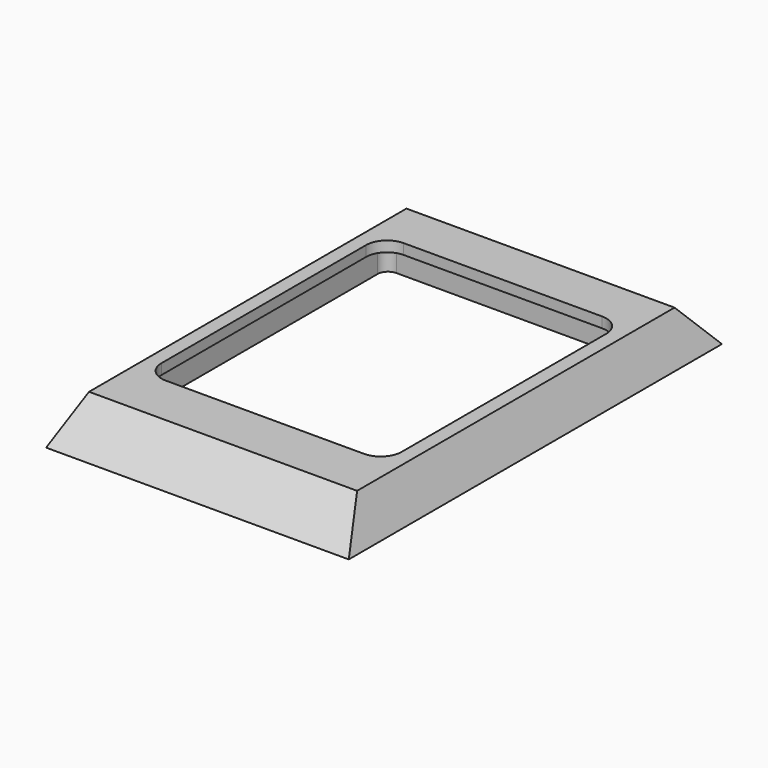
from build123d import *

# Parameters (mm, degrees)
F1_W        = 60
F1_H        = 93
F2_DEPTH    = 8
F3_T1_DEPTH = 147.142599219
F4_T1_DEPTH = 102.8305675527
F5_DEPTH    = 25
F6_DEPTH    = 6
F7_T1_DEPTH = 105.1482614058


# Not quite as in the source:
# - a fillet or chamfer that OpenCascade refuses, or shapes differently, is made with other operations: its cross-section is extruded or revolved along the edge and cut away or added


with BuildPart() as f2:
    # F1 (on Top) → F2 (new body)
    with BuildSketch(Plane.XY):
        Rectangle(F1_W, F1_H)
    extrude(amount=F2_DEPTH)

    # F3: chamfer of 4.325 x 10.4414736573 on 2 edges, made by hand

    # F3_s2 → F3_t1 (cut)
    with BuildSketch(Plane.XZ.offset(-73.5712996095)):
        Polygon((30, -2.4414736573), (25.675, 8), (30, 8), align=None)
        Polygon((-30, -2.4414736573), (-25.675, 8), (-30, 8), align=None)
    extrude(amount=F3_T1_DEPTH, mode=Mode.SUBTRACT)

    # F4: chamfer of 9 x 9.9955126335 on 1 edges, made by hand

    # F4_s2 → F4_t1 (cut)
    with BuildSketch(Plane.YZ.offset(-51.4152837764)):
        Polygon((37.5, 8), (46.5, -1.9955126335), (46.5, 8), align=None)
    extrude(amount=F4_T1_DEPTH, mode=Mode.SUBTRACT)

    # F0 (on Top) → F5 (cut)
    with BuildSketch(Plane.XY):
        with BuildLine():
            ThreePointArc((23, 24.5), (21.8284271247, 27.3284271247), (19, 28.5))
            Line((19, 28.5), (-19, 28.5))
            ThreePointArc((-19, 28.5), (-21.8284271247, 27.3284271247), (-23, 24.5))
            Line((-23, 24.5), (-23, -24.5))
            ThreePointArc((-23, -24.5), (-21.8284271247, -27.3284271247), (-19, -28.5))
            Line((-19, -28.5), (19, -28.5))
            ThreePointArc((19, -28.5), (21.8284271247, -27.3284271247), (23, -24.5))
            Line((23, -24.5), (23, 24.5))
        make_face()
    extrude(amount=F5_DEPTH, mode=Mode.SUBTRACT)

    # F0 (on Top) → F6 (cut)
    with BuildSketch(Plane.XY):
        with BuildLine():
            ThreePointArc((25.6034387499, 30.25), (25.0176523123, 31.6642135624), (23.6034387499, 32.25))
            Line((23.6034387499, 32.25), (-23.3965612501, 32.25))
            ThreePointArc((-23.3965612501, 32.25), (-24.8107748125, 31.6642135624), (-25.3965612501, 30.25))
            Line((-25.3965612501, 30.25), (-25.3965612501, -35.75))
            ThreePointArc((-25.3965612501, -35.75), (-24.8107748125, -37.1642135624), (-23.3965612501, -37.75))
            Line((-23.3965612501, -37.75), (23.6034387499, -37.75))
            ThreePointArc((23.6034387499, -37.75), (25.0176523123, -37.1642135624), (25.6034387499, -35.75))
            Line((25.6034387499, -35.75), (25.6034387499, 30.25))
        make_face()
        with BuildLine():
            Line((-19, 28.5), (19, 28.5))
            ThreePointArc((19, 28.5), (21.8284271247, 27.3284271247), (23, 24.5))
            Line((23, 24.5), (23, -24.5))
            ThreePointArc((23, -24.5), (21.8284271247, -27.3284271247), (19, -28.5))
            Line((19, -28.5), (-19, -28.5))
            ThreePointArc((-19, -28.5), (-21.8284271247, -27.3284271247), (-23, -24.5))
            Line((-23, -24.5), (-23, 24.5))
            ThreePointArc((-23, 24.5), (-21.8284271247, 27.3284271247), (-19, 28.5))
        make_face(mode=Mode.SUBTRACT)
    extrude(amount=F6_DEPTH, mode=Mode.SUBTRACT)

    # F7: chamfer of 8 x 10.4258029827 on 1 edges, made by hand

    # F7_s2 → F7_t1 (cut)
    with BuildSketch(Plane.YZ.offset(-52.5741307029)):
        Polygon((-46.5, -2.4258029827), (-38.5, 8), (-46.5, 8), align=None)
    extrude(amount=F7_T1_DEPTH, mode=Mode.SUBTRACT)


solid = f2.part
